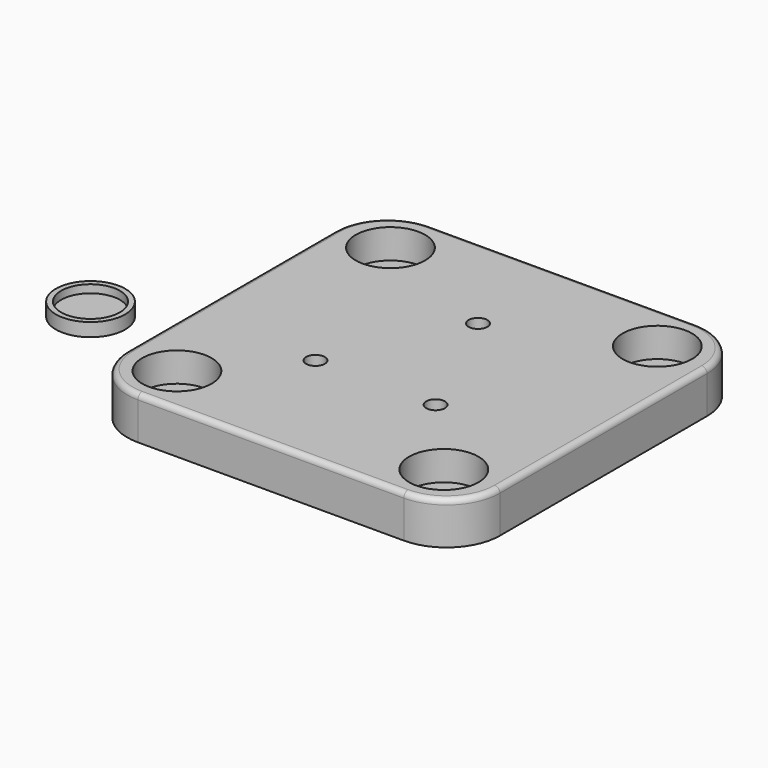
from build123d import *

# Parameters (mm, degrees)
F0_R     = 13
F0_R_2   = 8
F0_R_3   = 3.5
F1_DEPTH = 16
F2_DEPTH = 7
F3_DEPTH = 16
F4_R     = 2
F0_R_4   = 5.5
F5_DEPTH = 5
F0_R_5   = 11
F6_DEPTH = 2
F7_DEPTH = 5


# Not quite as in the source:
# - a feature names something its author has since deleted; it is built from what else it names


with BuildPart() as f1:
    # F0 (on Top) → F1 (new body)
    with BuildSketch(Plane.XY):
        with BuildLine():
            Line((99.8149545762, 18.5), (0.1850454238, 18.5))
            ThreePointArc((0.1850454238, 18.5), (-13.9570902, 12.6421356237), (-19.8149545762, -1.5))
            Line((-19.8149545762, -1.5), (-19.8149545762, -98.5))
            ThreePointArc((-19.8149545762, -98.5), (-13.9570902, -112.6421356237), (0.1850454238, -118.5))
            Line((0.1850454238, -118.5), (99.8149545762, -118.5))
            ThreePointArc((99.8149545762, -118.5), (113.9570902, -112.6421356237), (119.8149545762, -98.5))
            Line((119.8149545762, -98.5), (119.8149545762, -1.5))
            ThreePointArc((119.8149545762, -1.5), (113.9570902, 12.6421356237), (99.8149545762, 18.5))
        make_face()
        with Locations((0, -100)):
            Circle(F0_R, mode=Mode.SUBTRACT)
        with Locations((100, -100)):
            Circle(F0_R, mode=Mode.SUBTRACT)
        with Locations((27.5, -69.5)):
            Circle(F0_R_2, mode=Mode.SUBTRACT)
        with Locations((72.5, -69.5)):
            Circle(F0_R_2, mode=Mode.SUBTRACT)
        Circle(F0_R, mode=Mode.SUBTRACT)
        with Locations((50, -21.5)):
            Circle(F0_R_2, mode=Mode.SUBTRACT)
        with Locations((100, 0)):
            Circle(F0_R, mode=Mode.SUBTRACT)
        with Locations((50, -21.5)):
            Circle(F0_R_2)
        with Locations((50, -21.5)):
            Circle(F0_R_3, mode=Mode.SUBTRACT)
        with Locations((72.5, -69.5)):
            Circle(F0_R_2)
        with Locations((72.5, -69.5)):
            Circle(F0_R_3, mode=Mode.SUBTRACT)
        with Locations((27.5, -69.5)):
            Circle(F0_R_2)
        with Locations((27.5, -69.5)):
            Circle(F0_R_3, mode=Mode.SUBTRACT)
        with Locations((50, -21.5)):
            Circle(F0_R_3)
        with Locations((72.5, -69.5)):
            Circle(F0_R_3)
        with Locations((27.5, -69.5)):
            Circle(F0_R_3)
    extrude(amount=F1_DEPTH)

    # F0 (on Top) → F2 (cut)
    with BuildSketch(Plane.XY):
        with Locations((72.5, -69.5)):
            Circle(F0_R_2)
        with Locations((72.5, -69.5)):
            Circle(F0_R_3, mode=Mode.SUBTRACT)
        with Locations((27.5, -69.5)):
            Circle(F0_R_2)
        with Locations((27.5, -69.5)):
            Circle(F0_R_3, mode=Mode.SUBTRACT)
        with Locations((50, -21.5)):
            Circle(F0_R_2)
        with Locations((50, -21.5)):
            Circle(F0_R_3, mode=Mode.SUBTRACT)
    extrude(amount=F2_DEPTH, mode=Mode.SUBTRACT)

    # F0 (on Top) → F3 (cut, through all)
    with BuildSketch(Plane.XY):
        with Locations((27.5, -69.5)):
            Circle(F0_R_3)
        with Locations((72.5, -69.5)):
            Circle(F0_R_3)
        with Locations((50, -21.5)):
            Circle(F0_R_3)
    extrude(amount=F3_DEPTH, mode=Mode.SUBTRACT)

    # F4
    f4_edges = [f1.edges().sort_by_distance(p)[0] for p in [
        (119.814955, -50, 16),
    ]]
    fillet(f4_edges, radius=F4_R)

    # F0 (on Top) → F5 (join)
    with BuildSketch(Plane.XY):
        with Locations((100, 0)):
            Circle(F0_R)
        with Locations((100, 0)):
            Circle(F0_R_4, mode=Mode.SUBTRACT)
        with Locations((100, -100)):
            Circle(F0_R)
        with Locations((100, -100)):
            Circle(F0_R_4, mode=Mode.SUBTRACT)
        with Locations((0, -100)):
            Circle(F0_R)
        with Locations((0, -100)):
            Circle(F0_R_4, mode=Mode.SUBTRACT)
        Circle(F0_R)
        Circle(F0_R_4, mode=Mode.SUBTRACT)
    extrude(amount=F5_DEPTH)


with BuildPart() as f6:
    # F0 (on Top) → F6 (new body)
    with BuildSketch(Plane.XY):
        with Locations((-60.3785477579, -64.9964138865)):
            Circle(F0_R)
        with Locations((-60.3785477579, -64.9964138865)):
            Circle(F0_R_5, mode=Mode.SUBTRACT)
        with Locations((-60.3785477579, -64.9964138865)):
            Circle(F0_R_5)
    extrude(amount=F6_DEPTH)

    # F0 (on Top) → F7 (join)
    with BuildSketch(Plane.XY):
        with Locations((-60.3785477579, -64.9964138865)):
            Circle(F0_R)
        with Locations((-60.3785477579, -64.9964138865)):
            Circle(F0_R_5, mode=Mode.SUBTRACT)
    extrude(amount=F7_DEPTH)


solid = Compound([f1.part, f6.part])
